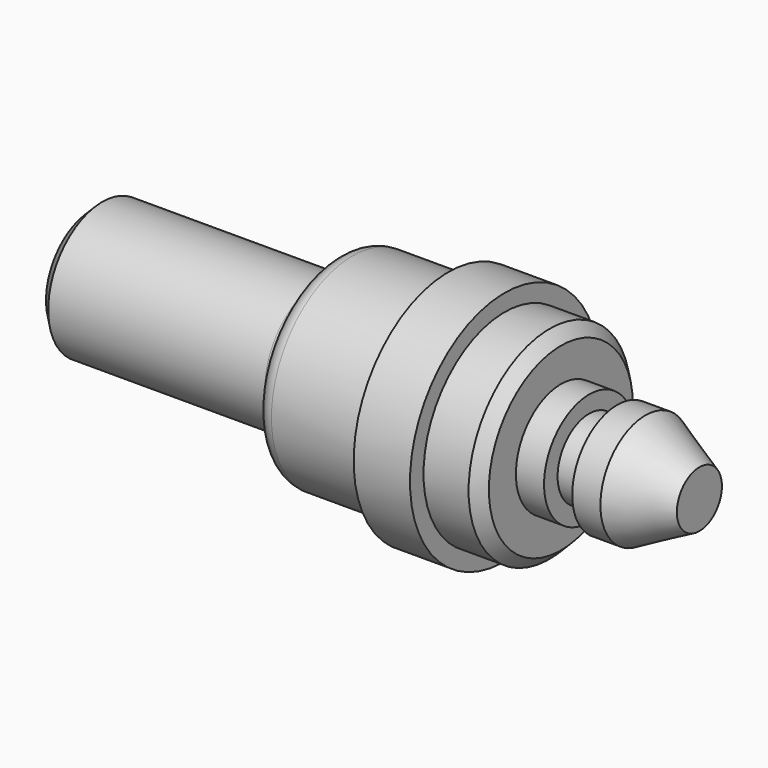
from build123d import *

# Parameters (mm, degrees)
F2_R    = 2.99999
F3_SIZE = 2


# Not quite as in the source:
# - a fillet or chamfer is up to 0.001 mm smaller than in the source, because OpenCascade refuses the exact size


with BuildPart() as f1:
    # F0 (on Top) → F1 (revolve)
    with BuildSketch(Plane.XY):
        Polygon((-62.0045285772, 2), (-62.0045285772, -10), (45.9954714228, -10), (45.9954714228, -5), (36.4192584626, 0), (31.4192584626, 0), (31.4192584626, -3), (26.4192584626, -3), (26.4192584626, 0), (21.4192584626, 0), (21.4192584626, 8), (11.4192584626, 8), (11.4192584626, 11), (1.4192584626, 11), (1.4192584626, 8), (-18.5807415374, 8), (-18.5807415374, 2), align=None)
    revolve(axis=Axis((-8.0045285772, -10, 0), (1, 0, 0)))

    # F2 (radius 3 in the source; OpenCascade refuses exactly that, so slightly less here)
    f2_edges = [f1.edges().sort_by_distance(p)[0] for p in [
        (-18.580742, -28, 0),
        (-18.580742, -22, 0),
    ]]
    fillet(f2_edges, radius=F2_R)

    # F3
    f3_edges = [f1.edges().sort_by_distance(p)[0] for p in [
        (21.419258, -28, 0),
        (-62.004529, -22, 0),
    ]]
    chamfer(f3_edges, length=F3_SIZE)


solid = f1.part
